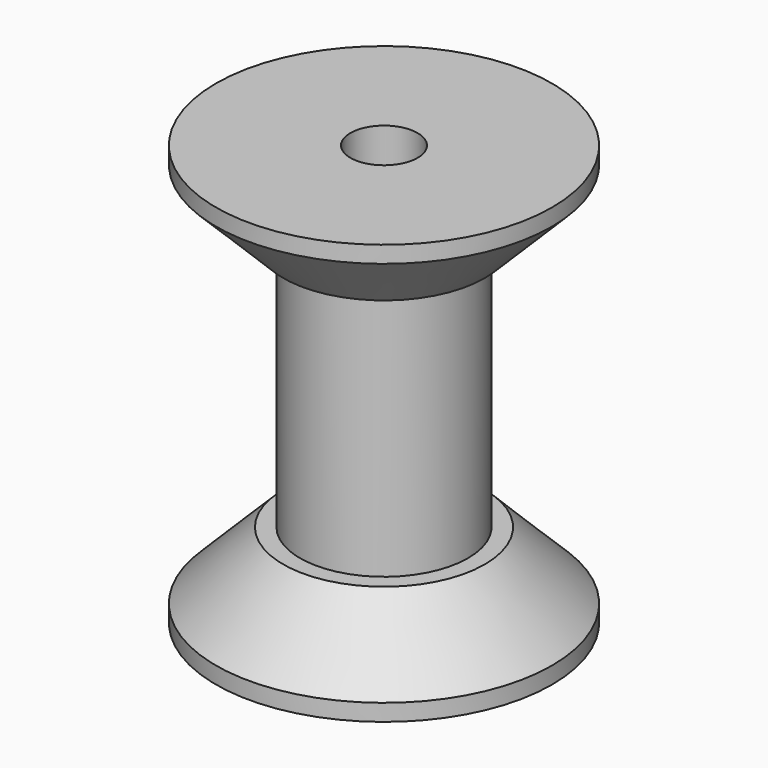
from build123d import *

# Parameters (mm, degrees)
F0_R     = 12.7
F1_DEPTH = 6.35
F2_R     = 6.35
F3_DEPTH = 25.4
F5_R     = 12.7
F6_DEPTH = 6.35
F7_R     = 2.54
F8_DEPTH = 31.75
F9_SIZE  = 5.08


# Not quite as in the source:
# - a pattern or mirror of a feature is missing from the dataset's text; its kind, count and spacing are read off the source's solid


with BuildPart() as f1:
    # F0 (on Top) → F1 (new body)
    with BuildSketch(Plane.XY):
        Circle(F0_R)
    extrude(amount=F1_DEPTH)


with BuildPart() as f1_copies_1:
    # F1_copies: instance of F1
    add(f1.part.mirror(Plane.XY.offset(15.875)))


with BuildPart() as f1_1:
    add(f1.part)

    add(f1_copies_1.part)  # F3 merges F1_copies_1
    # F2 (on Top) → F3 (join)
    with BuildSketch(Plane.XY):
        Circle(F2_R)
    extrude(amount=F3_DEPTH)

    # F5 (on face) → F6 (join)
    with BuildSketch(Plane.XY.offset(25.4)):
        Circle(F5_R)
    extrude(amount=F6_DEPTH)

    # F7 (on face) → F8 (cut)
    with BuildSketch(Plane.XY.offset(31.75)):
        Circle(F7_R)
    extrude(amount=-F8_DEPTH, mode=Mode.SUBTRACT)

    # F9
    f9_edges = [f1_1.edges().sort_by_distance(p)[0] for p in [
        (-12.7, 0, 25.4),
        (-12.7, 0, 6.35),
    ]]
    chamfer(f9_edges, length=F9_SIZE)


solid = f1_1.part
